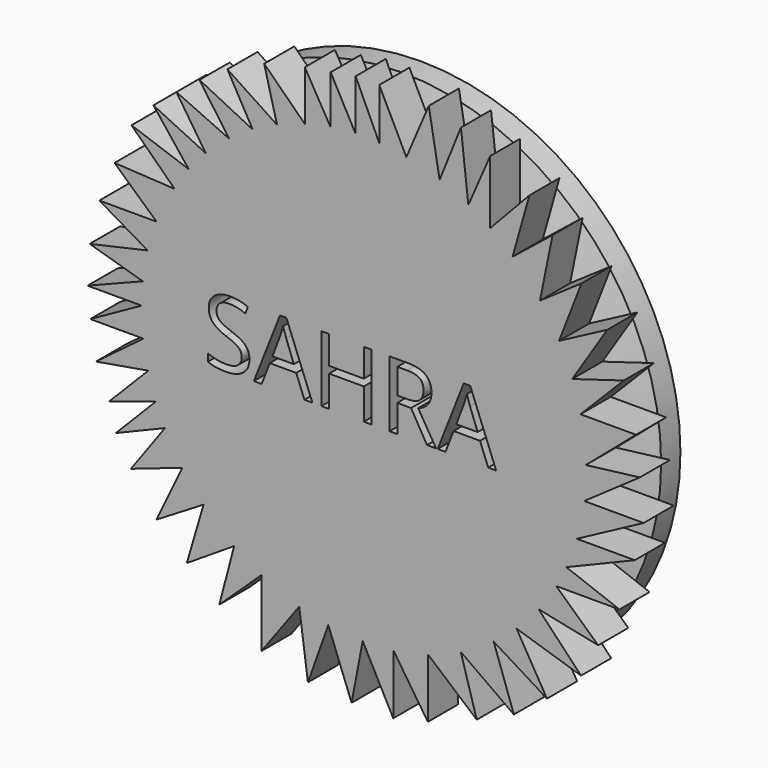
from build123d import *

# Parameters (mm, degrees)
F0_W         = 15.0114
F0_H         = 14.1830341901
F0_W_2       = 7.2136
F0_H_2       = 22.4835798259
F2_R         = 1.5875
F3_SIZE      = 0.79375
F4_SIZE2     = 6.35
F4_SIZE      = 1.5748
F6_DEPTH     = 6.35
F7_TEXT_SIZE = 15.5744970673
F8_DEPTH     = 5.08
F9_R         = 5.08


# Not quite as in the source:
# - Text() gives the source's letters only with a copy of the font that has no kerning and outlines rounded to 1/6400 em; it was checked with that copy


with BuildPart() as f1:
    # F0 (on Right) → F1 (revolve)
    with BuildSketch(Plane.YZ):
        with Locations((5.3087373331, -14.2041580942)):
            Rectangle(F0_W, F0_H)
        with Locations((-5.8037626669, -14.2041580942)):
            Rectangle(F0_W_2, F0_H)
        with Locations((-5.8037626669, -32.5374651022)):
            Rectangle(F0_W_2, F0_H_2)
    revolve(axis=Axis((0, 18.1947540087, 0), (0, 1, 0)))

    # F2
    f2_edges = [f1.edges().sort_by_distance(p)[0] for p in [
        (0, -2.196963, 21.295675),
    ]]
    fillet(f2_edges, radius=F2_R)

    # F3
    f3_edges = [f1.edges().sort_by_distance(p)[0] for p in [
        (0, 12.814437, 21.295675),
    ]]
    chamfer(f3_edges, length=F3_SIZE)

    # F4
    f4_edges = [f1.edges().sort_by_distance(p)[0] for p in [
        (0, -9.410563, 43.779255),
        (0, -2.196963, 43.779255),
    ]]
    f4_side = f1.faces().sort_by_distance((0, -5.803763, 43.779255))[0]
    chamfer(f4_edges, length=F4_SIZE, length2=F4_SIZE2, reference=f4_side)

    # F5 (on face) → F6 (join)
    with BuildSketch(Plane.XZ.offset(9.4105626669)):
        Polygon((-22.696380741, 29.7627860297), (-31.5618552268, 33.7978489697), (-26.6145392206, 26.3175879037), (-35.4385823011, 30.5677186698), (-29.5037029228, 23.0321654396), (-39.1351729631, 26.4044106007), (-31.8752378225, 19.3291287869), (-41.9888794422, 19.8935642838), (-34.9193755739, 13.4753976017), (-44.5534735918, 13.4753976017), (-36.4001131606, 8.7167019501), (-46.1747087538, 6.5206927247), (-37.2277001301, 3.8791073737), (-46.5395227076, 0.2007674251), (-37.4287165614, 0.2007674251), (-46.0751588329, -4.6051374351), (-37.1448763654, -4.6051374351), (-45.1203286648, -10.5971936136), (-36.3099534916, -9.0849550593), (-42.9254546762, -15.81521146), (-35.0134893374, -13.2289340242), (-41.7767092586, -20.1162956655), (-33.5010257201, -16.6922259359), (-39.2341427505, -24.5972909033), (-30.5527686181, -21.6212270874), (-34.9266529083, -30.7327434421), (-26.9923590742, -25.9299379599), (-29.8064574599, -35.5097055435), (-21.8394795726, -30.3971423491), (-24.3302732706, -39.8891754448), (-17.2540433705, -33.2151639822), (-17.2540433705, -44.4924049079), (-10.8719548077, -35.8154956639), (-9.4040138647, -46.5713590384), (-5.9724703897, -36.9496783266), (-2.0475925412, -47.2171828151), (-0.175778332, -37.4288422606), (4.9754025578, -47.2326587704), (4.9754025578, -37.0970955788), (10.8054888869, -45.8705916614), (10.8054888869, -35.8356043748), (19.0439000726, -42.8679063916), (16.3501440553, -33.6693023445), (25.2998489887, -40.0562286377), (21.9003674813, -30.3533035299), (30.885418877, -35.8894094825), (25.7503731495, -27.1637150194), (36.622684449, -30.608240515), (29.4668049751, -23.0793530142), (39.5078137517, -25.1674614847), (32.4329394923, -18.682975322), (43.092764914, -18.682975322), (34.1486646787, -15.3237668887), (45.6794271609, -10.5363345907), (35.9156621043, -10.5363345907), (47.1741751785, -4.5291274876), (37.1542209607, -4.5291274876), (46.5385578573, 2.0259069279), (37.4184992982, 0.8972409161), (45.8855362991, 8.1386118317), (36.5337122183, 8.1386118317), (43.8198372722, 15.5148757622), (35.13137933, 12.9126030439), (41.0425961018, 22.137388587), (32.904731868, 17.8389391974), (36.6931408644, 27.6000387967), (29.7004223929, 22.7779288057), (31.8169295788, 33.1723019481), (25.0812474996, 27.7827312347), (27.9109962285, 37.8064289689), (21.2944149971, 30.7814395525), (21.2944149971, 41.4811894298), (17.6301024781, 33.0170958385), (16.3774080575, 44.1186800599), (12.7857492829, 35.1777450424), (10.9621146694, 45.5788075924), (7.181599386, 36.7338231233), (2.617625427, 45.9594504495), (2.617625427, 37.3376106375), (-1.3658080232, 45.959450398), (-1.3658080232, 37.4043272823), (-5.5709413984, 45.1842073766), (-5.5709413984, 37.0123458177), (-9.9309971909, 44.5123319152), (-9.9309971909, 36.0877323448), (-16.7754907161, 42.8068004549), (-14.6193910426, 34.456095782), (-22.9774229228, 39.9642474949), (-18.7153591286, 32.4142632753), (-27.6805534959, 36.8632860482), align=None)
    extrude(amount=F6_DEPTH)

    # F7 (on face) → F8 (cut)
    with BuildSketch(Plane.XZ.offset(15.7605626669)):
        with Locations((-27.0626470447, -4.841722548)):
            Text('SAHRA', F7_TEXT_SIZE, font='Open Sans', text_align=(TextAlign.LEFT, TextAlign.BOTTOM))
    extrude(amount=-F8_DEPTH, mode=Mode.SUBTRACT)

    # F9
    f9_edges = [f1.edges().sort_by_distance(p)[0] for p in [
        (0, 12.814437, 7.112641),
    ]]
    fillet(f9_edges, radius=F9_R)


solid = f1.part
